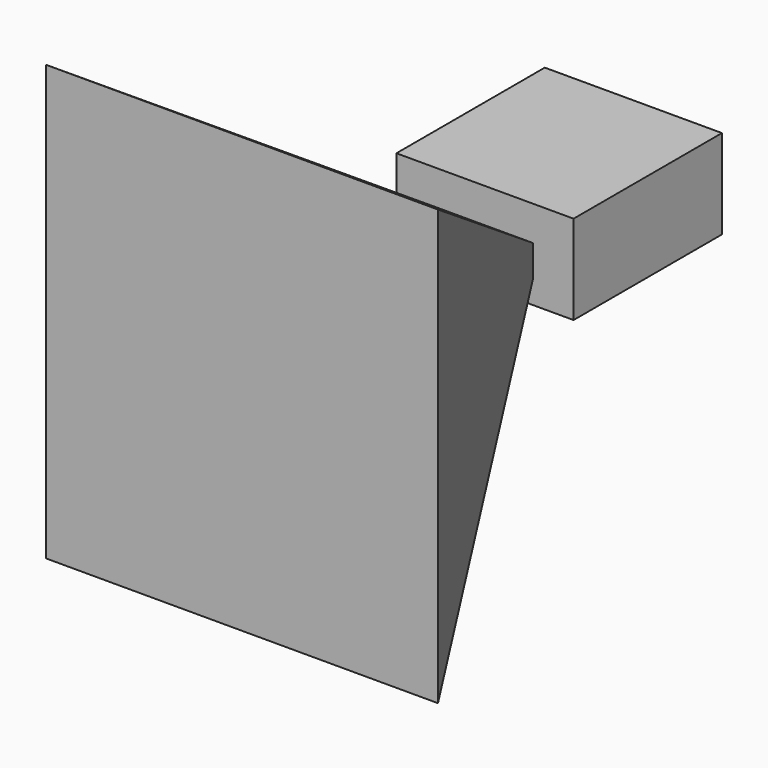
from build123d import *

# Parameters (mm, degrees)
F1_W     = 58.32
F1_H     = 61.06
F1_R     = 1.5
F2_DEPTH = 29.39
F8_W     = 129.0165177132
F8_H     = 143.0771122391
F3_W     = 31.47
F3_H     = 10.7


with BuildPart() as f2:
    # F1 (on offset) → F2 (new body)
    with BuildSketch(Plane.XY.offset(-12.64)):
        with Locations((0, 30.53)):
            Rectangle(F1_W, F1_H)
        with Locations((15.73, 16.46)):
            Circle(F1_R, mode=Mode.SUBTRACT)
        with Locations((-15.77, 46.69)):
            Circle(F1_R, mode=Mode.SUBTRACT)
        with Locations((-15.77, 46.69)):
            Circle(F1_R)
        with Locations((15.73, 16.46)):
            Circle(F1_R)
    extrude(amount=F2_DEPTH)

    # F8 (on offset) → F9 section 0
    with BuildSketch(Plane.XZ.offset(100)):
        Rectangle(F8_W, F8_H)
    # F3 (on face) → F9 section 1
    with BuildSketch(Plane.XZ):
        Rectangle(F3_W, F3_H)
    loft()


solid = f2.part
